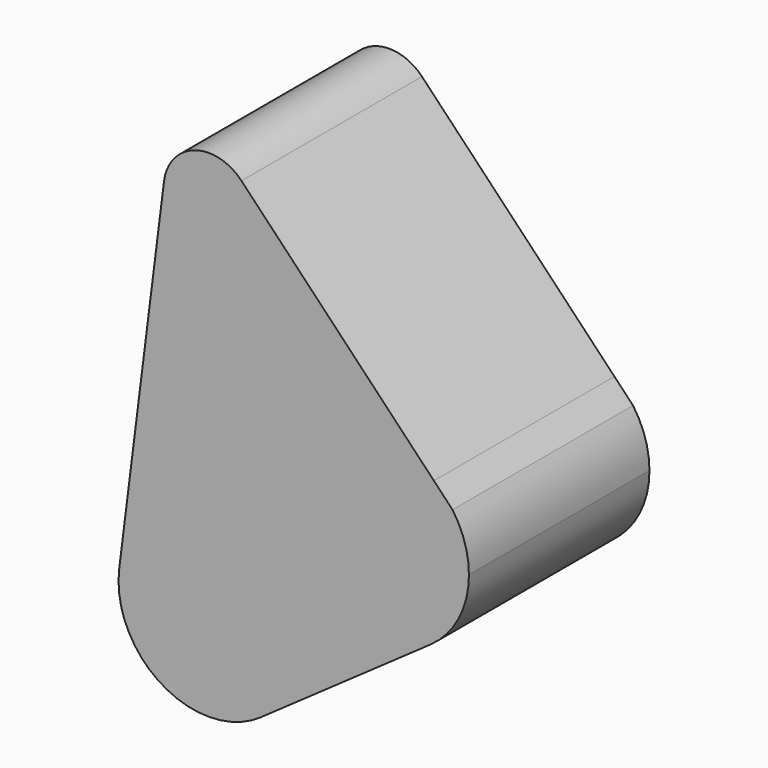
from build123d import *

# Parameters (mm, degrees)
F1_DEPTH = 25


# Not quite as in the source:
# - a feature names something its author has since deleted; it is built from what else it names


with BuildPart() as f1:
    # F0 (on Front) → F1 (new body)
    with BuildSketch(Plane.XZ):
        with BuildLine():
            ThreePointArc((5, 40), (4.4370598373, 37.6951138857), (2.875, 35.909232957))
            Line((2.875, 35.909232957), (13.0675283977, 21.406534086))
            ThreePointArc((13.0675283977, 21.406534086), (19.0462821804, 23.222383243), (24.9357240699, 21.1349735599))
            Line((24.9357240699, 21.1349735599), (3.6154854181, 43.4537320671))
            ThreePointArc((3.6154854181, 43.4537320671), (4.6409819592, 41.8604532928), (5, 40))
        make_face()
        with BuildLine():
            ThreePointArc((-9.9215674165, 1.25), (-6.6143782777, 7.5), (0, 10))
            Line((0, 10), (0, 35))
            ThreePointArc((0, 35), (-3.75, 36.6928108612), (-4.9607837082, 40.625))
            Line((-4.9607837082, 40.625), (-9.9215674165, 1.25))
        make_face()
        with BuildLine():
            Line((0, 35), (0, 10))
            ThreePointArc((0, 10), (4.6097722286, 8.8741196746), (8.181534086, 5.75))
            Line((8.181534086, 5.75), (10.6359943118, 7.475))
            ThreePointArc((10.6359943118, 7.475), (8.9664461732, 14.9443542409), (13.0675283977, 21.406534086))
            Line((13.0675283977, 21.406534086), (2.875, 35.909232957))
            ThreePointArc((2.875, 35.909232957), (1.5076744982, 35.2327242992), (0, 35))
        make_face()
        with BuildLine():
            Line((0, 40), (0, 35))
            ThreePointArc((0, 35), (1.5076744982, 35.2327242992), (2.875, 35.909232957))
            Line((2.875, 35.909232957), (0, 40))
        make_face()
        with BuildLine():
            Line((5.75, -8.181534086), (0, 0))
            Line((0, 0), (0, 10))
            ThreePointArc((0, 10), (-6.6143782777, 7.5), (-9.9215674165, 1.25))
            ThreePointArc((-9.9215674165, 1.25), (-5.1564476611, -8.5680247151), (5.75, -8.181534086))
        make_face()
        with BuildLine():
            Line((0, 10), (0, 0))
            Line((0, 0), (8.181534086, 5.75))
            ThreePointArc((8.181534086, 5.75), (4.6097722286, 8.8741196746), (0, 10))
        make_face()
        with BuildLine():
            Line((18.8175283977, 13.225), (24.5675283977, 5.043465914))
            ThreePointArc((24.5675283977, 5.043465914), (27.6916480724, 8.6152277714), (28.8175283977, 13.225))
            ThreePointArc((28.8175283977, 13.225), (28.3520797994, 16.2403489964), (26.9990624837, 18.975))
            Line((26.9990624837, 18.975), (18.8175283977, 13.225))
        make_face()
        with BuildLine():
            ThreePointArc((13.0675283977, 21.406534086), (8.9664461732, 14.9443542409), (10.6359943118, 7.475))
            Line((10.6359943118, 7.475), (18.8175283977, 13.225))
            Line((18.8175283977, 13.225), (13.0675283977, 21.406534086))
        make_face()
        with BuildLine():
            Line((13.0675283977, 21.406534086), (18.8175283977, 13.225))
            Line((18.8175283977, 13.225), (26.9990624837, 18.975))
            Line((26.9990624837, 18.975), (24.9357240699, 21.1349735599))
            ThreePointArc((24.9357240699, 21.1349735599), (19.0462821804, 23.222383243), (13.0675283977, 21.406534086))
        make_face()
        with BuildLine():
            Line((10.6359943118, 7.475), (8.181534086, 5.75))
            ThreePointArc((8.181534086, 5.75), (9.5345514016, 3.0153489964), (10, 0))
            ThreePointArc((10, 0), (8.8741196746, -4.6097722286), (5.75, -8.181534086))
            Line((5.75, -8.181534086), (24.5675283977, 5.043465914))
            ThreePointArc((24.5675283977, 5.043465914), (17.0981741569, 3.3739177755), (10.6359943118, 7.475))
        make_face()
        with BuildLine():
            Line((8.181534086, 5.75), (0, 0))
            Line((0, 0), (5.75, -8.181534086))
            ThreePointArc((5.75, -8.181534086), (8.8741196746, -4.6097722286), (10, 0))
            ThreePointArc((10, 0), (9.5345514016, 3.0153489964), (8.181534086, 5.75))
        make_face()
        with BuildLine():
            Line((18.8175283977, 13.225), (10.6359943118, 7.475))
            ThreePointArc((10.6359943118, 7.475), (17.0981741569, 3.3739177755), (24.5675283977, 5.043465914))
            Line((24.5675283977, 5.043465914), (18.8175283977, 13.225))
        make_face()
        with BuildLine():
            ThreePointArc((-4.9607837082, 40.625), (-3.75, 36.6928108612), (0, 35))
            Line((0, 35), (0, 40))
            Line((0, 40), (2.875, 35.909232957))
            ThreePointArc((2.875, 35.909232957), (4.4370598373, 37.6951138857), (5, 40))
            ThreePointArc((5, 40), (4.6409819592, 41.8604532928), (3.6154854181, 43.4537320671))
            ThreePointArc((3.6154854181, 43.4537320671), (-1.566169898, 44.7483799185), (-4.9607837082, 40.625))
        make_face()
    extrude(amount=F1_DEPTH)


solid = f1.part
